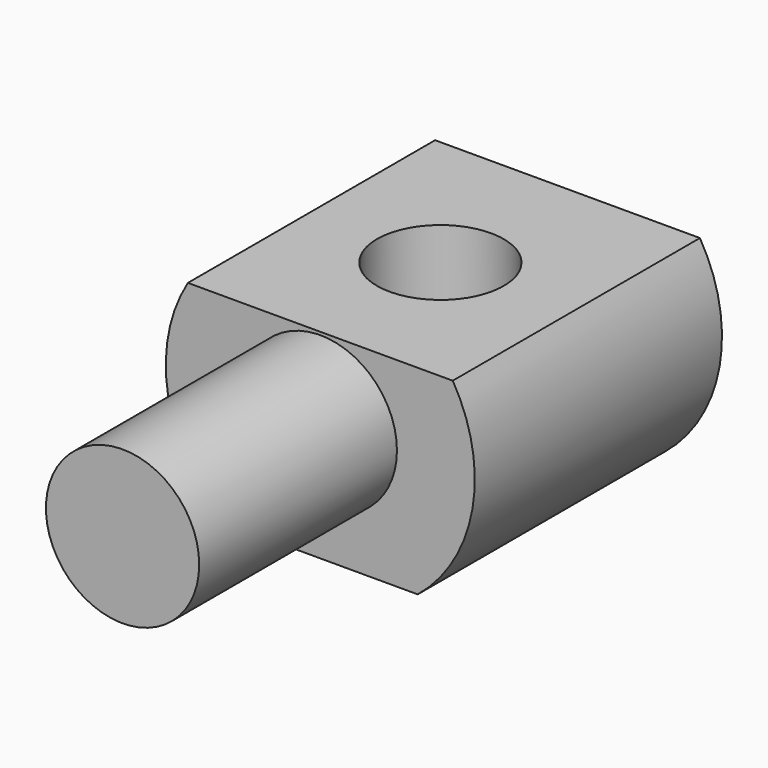
from build123d import *

# Parameters (mm, degrees)
F1_DEPTH = 22.225
F2_R     = 5.5118
F3_DEPTH = 17.78
F5_D     = 9.1186


# Not quite as in the source:
# - ends of sketch curves that miss each other by under 0.0002 mm in the source are joined


with BuildPart() as f1:
    # F0 (on Front) → F1 (new body)
    with BuildSketch(Plane.XZ):
        with BuildLine():
            ThreePointArc((7.0042338121, -8.6271875461), (10.9449391879, -1.9224886016), (9.5250001177, 5.7238124539))
            Line((9.5250001177, 5.7238124539), (-9.5250001177, 5.7238124539))
            ThreePointArc((-9.5250001177, 5.7238124539), (-10.9449391879, -1.9224886016), (-7.0042338121, -8.6271875461))
            Line((-7.0042338121, -8.6271875461), (7.0042338121, -8.6271875461))
        make_face()
    extrude(amount=F1_DEPTH)

    # F2 (on face) → F3 (join)
    with BuildSketch(Plane.XZ.offset(22.225)):
        Circle(F2_R)
    extrude(amount=F3_DEPTH)

    # F5 (through all)
    with Locations(Plane(origin=(0, 0, -8.6271875461), x_dir=(1, 0, 0), z_dir=(0, 0, -1))):
        with Locations((0, 11.43)):
            Hole(F5_D / 2)


solid = f1.part
